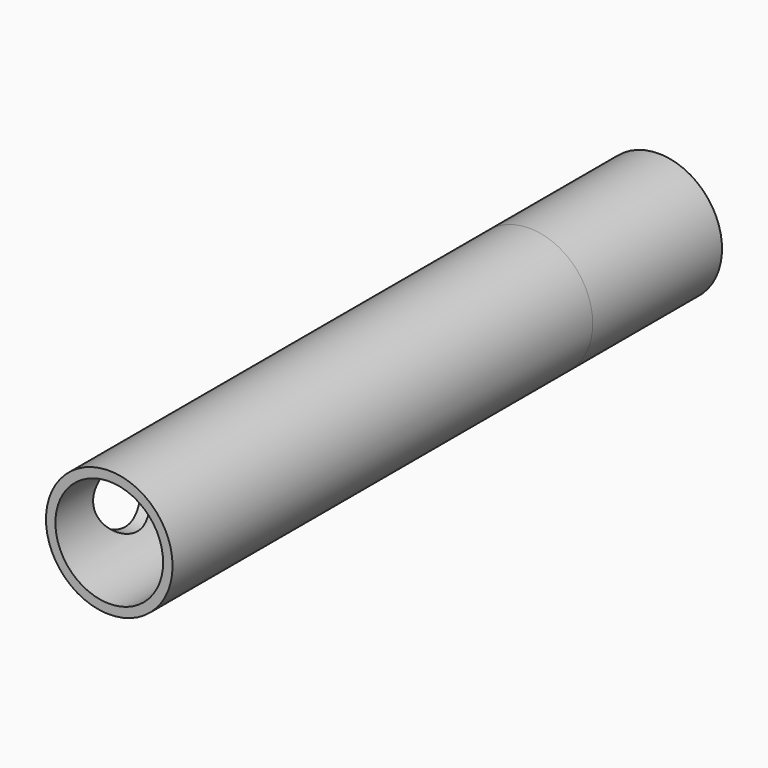
from build123d import *

# Parameters (mm, degrees)
F3_R      = 4.7
F4_DEPTH  = 29
F8_DEPTH  = 29
F6_R      = 4.7
F6_R_2    = 4
F9_DEPTH  = 10
F7_R      = 4.7
F7_R_2    = 4
F10_DEPTH = 12
F11_R     = 2.75
F12_DEPTH = 4.701


# Not quite as in the source:
# - ends of sketch curves that miss each other by under 0.0002 mm in the source are joined


with BuildPart() as f4:
    # F3 (on Front) → F4 (new body)
    with BuildSketch(Plane.XZ):
        Circle(F3_R)
    extrude(amount=F4_DEPTH)

    # F5 (on face) → F8 (cut, through all)
    with BuildSketch(Plane.XZ.offset(29)):
        with BuildLine():
            Line((-1.25, -3.8), (0, -3.8))
            Line((0, -3.8), (1.25, -3.8))
            Line((1.25, -3.8), (1.25, -3.7))
            ThreePointArc((1.25, -3.7), (1.3085786438, -3.5585786438), (1.45, -3.5))
            Line((1.45, -3.5), (2, -3.5))
            Line((2, -3.5), (2, -3.05))
            ThreePointArc((2, -3.05), (2.0585786438, -2.9085786438), (2.2, -2.85))
            Line((2.2, -2.85), (3.15, -2.85))
            Line((3.15, -2.85), (3.15, -2.15))
            Line((3.15, -2.15), (2.2, -2.15))
            ThreePointArc((2.2, -2.15), (2.0585786438, -2.0914213562), (2, -1.95))
            Line((2, -1.95), (2, -1.887459))
            ThreePointArc((2, -1.887459), (2.1033535752, -1.771554046), (2.2, -1.65))
            Line((2.2, -1.65), (3.75, -1.65))
            Line((3.75, -1.65), (3.75, 0))
            Line((3.75, 0), (3.75, 1.65))
            Line((3.75, 1.65), (2.2, 1.65))
            ThreePointArc((2.2, 1.65), (2.1033535752, 1.771554046), (1.9999998047, 1.8874588157))
            Line((1.9999998047, 1.8874588157), (2, 1.95))
            ThreePointArc((2, 1.95), (2.0585786438, 2.0914213562), (2.2, 2.15))
            Line((2.2, 2.15), (3.15, 2.15))
            Line((3.15, 2.15), (3.15, 2.85))
            Line((3.15, 2.85), (2.2, 2.85))
            ThreePointArc((2.2, 2.85), (2.0585786438, 2.9085786438), (2, 3.05))
            Line((2, 3.05), (2, 3.5))
            Line((2, 3.5), (1.45, 3.5))
            ThreePointArc((1.45, 3.5), (1.3085786438, 3.5585786438), (1.25, 3.7))
            Line((1.25, 3.7), (1.25, 3.8))
            Line((1.25, 3.8), (0, 3.8))
            Line((0, 3.8), (-1.25, 3.8))
            Line((-1.25, 3.8), (-1.25, 3.7))
            ThreePointArc((-1.25, 3.7), (-1.3085786438, 3.5585786438), (-1.45, 3.5))
            Line((-1.45, 3.5), (-2, 3.5))
            Line((-2, 3.5), (-2, 3.05))
            ThreePointArc((-2, 3.05), (-2.0585786438, 2.9085786438), (-2.2, 2.85))
            Line((-2.2, 2.85), (-3.15, 2.85))
            Line((-3.15, 2.85), (-3.15, 2.15))
            Line((-3.15, 2.15), (-2.2, 2.15))
            ThreePointArc((-2.2, 2.15), (-2.0585786438, 2.0914213562), (-2, 1.95))
            Line((-2, 1.95), (-2, 1.887459))
            ThreePointArc((-2, 1.887459), (-2.1033535752, 1.771554046), (-2.2, 1.65))
            Line((-2.2, 1.65), (-3.75, 1.65))
            Line((-3.75, 1.65), (-3.75, 0))
            Line((-3.75, 0), (-3.75, -1.65))
            Line((-3.75, -1.65), (-2.2, -1.65))
            ThreePointArc((-2.2, -1.65), (-2.1033535752, -1.771554046), (-1.9999998047, -1.8874588157))
            Line((-1.9999998047, -1.8874588157), (-2, -1.95))
            ThreePointArc((-2, -1.95), (-2.0585786438, -2.0914213562), (-2.2, -2.15))
            Line((-2.2, -2.15), (-3.15, -2.15))
            Line((-3.15, -2.15), (-3.15, -2.85))
            Line((-3.15, -2.85), (-2.2, -2.85))
            ThreePointArc((-2.2, -2.85), (-2.0585786438, -2.9085786438), (-2, -3.05))
            Line((-2, -3.05), (-2, -3.5))
            Line((-2, -3.5), (-1.45, -3.5))
            ThreePointArc((-1.45, -3.5), (-1.3085786438, -3.5585786438), (-1.25, -3.7))
            Line((-1.25, -3.7), (-1.25, -3.8))
        make_face()
    extrude(amount=-F8_DEPTH, mode=Mode.SUBTRACT)

    # F6 (on face) → F9 (join)
    with BuildSketch(Plane.XZ.offset(29)):
        Circle(F6_R)
        Circle(F6_R_2, mode=Mode.SUBTRACT)
    extrude(amount=F9_DEPTH)

    # F7 (on face) → F10 (join)
    with BuildSketch(Plane(origin=(0, 0, 0), x_dir=(-1, 0, 0), z_dir=(0, 1, 0))):
        Circle(F7_R)
        Circle(F7_R_2, mode=Mode.SUBTRACT)
    extrude(amount=F10_DEPTH)

    # F11 (on Right) → F12 (cut, through all)
    with BuildSketch(Plane.YZ):
        with Locations((-32.75, 0)):
            Circle(F11_R)
    extrude(amount=-F12_DEPTH, mode=Mode.SUBTRACT)


solid = f4.part
